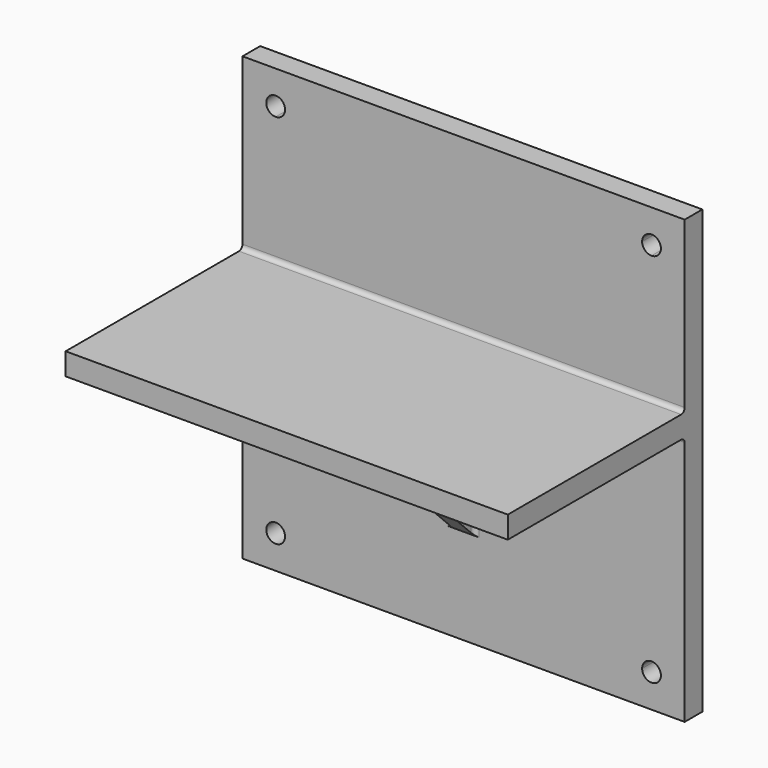
from build123d import *

# Parameters (mm, degrees)
F0_W         = 100
F0_H         = 10
F1_DEPTH     = 200
F2_W         = 10
F2_H         = 70
F3_DEPTH     = 70
F5_DEPTH     = 70
F7_DEPTH     = 20
F8_T1_DEPTH  = 200
F8_T3_DEPTH  = 93
F8_T5_DEPTH  = 93
F8_S9_W      = 2
F8_S9_H      = 2
F8_T10_DEPTH = 2
F8_S15_W     = 2
F8_S15_H     = 2
F8_T16_DEPTH = 2
F8_T22_DEPTH = 73
F8_T27_DEPTH = 73
F8_T32_DEPTH = 73
F8_T37_DEPTH = 73


# Not quite as in the source:
# - a fillet or chamfer that OpenCascade refuses, or shapes differently, is made with other operations: its cross-section is extruded or revolved along the edge and cut away or added


with BuildPart() as f1:
    # F0 (on Right) → F1 (new body)
    with BuildSketch(Plane.YZ):
        Polygon((5, -100), (5, 100), (-5, 100), (-5, 23.2), (-5, 13.2), (-5, -100), align=None)
        with Locations((-55, 18.2)):
            Rectangle(F0_W, F0_H)
    extrude(amount=F1_DEPTH)

    # F2 (on face) → F3 (join)
    with BuildSketch(Plane.XZ.offset(5)):
        with Locations((100, -21.8)):
            Rectangle(F2_W, F2_H)
    extrude(amount=F3_DEPTH)

    # F4 (on face) → F5 (cut)
    with BuildSketch(Plane(origin=(95, 0, 0), x_dir=(0, -1, 0), z_dir=(-1, 0, 0))):
        Polygon((75, -56.8), (75, 13.2), (5, -56.8), align=None)
    extrude(amount=-F5_DEPTH, mode=Mode.SUBTRACT)

    # F6 (on face) → F7 (cut)
    with BuildSketch(Plane.XZ.offset(5)):
        with BuildLine():
            Line((15, 80.75), (15, 85))
            Line((15, 85), (19.25, 85))
            ThreePointArc((19.25, 85), (11.99479618, 88.00520382), (15, 80.75))
        make_face()
        with BuildLine():
            Line((19.25, 85), (15, 85))
            Line((15, 85), (15, 80.75))
            ThreePointArc((15, 80.75), (18.00520382, 81.99479618), (19.25, 85))
        make_face()
        with BuildLine():
            ThreePointArc((189.25, 85), (185, 89.25), (180.75, 85))
            Line((180.75, 85), (185, 85))
            Line((185, 85), (185, 80.75))
            ThreePointArc((185, 80.75), (188.00520382, 81.99479618), (189.25, 85))
        make_face()
        with BuildLine():
            Line((185, 85), (180.75, 85))
            ThreePointArc((180.75, 85), (181.99479618, 81.99479618), (185, 80.75))
            Line((185, 80.75), (185, 85))
        make_face()
        with BuildLine():
            ThreePointArc((189.25, -85), (188.00520382, -81.99479618), (185, -80.75))
            Line((185, -80.75), (185, -85))
            Line((185, -85), (180.75, -85))
            ThreePointArc((180.75, -85), (185, -89.25), (189.25, -85))
        make_face()
        with BuildLine():
            Line((185, -85), (185, -80.75))
            ThreePointArc((185, -80.75), (181.99479618, -81.99479618), (180.75, -85))
            Line((180.75, -85), (185, -85))
        make_face()
        with BuildLine():
            Line((15, -85), (15, -80.75))
            ThreePointArc((15, -80.75), (11.99479618, -88.00520382), (19.25, -85))
            Line((19.25, -85), (15, -85))
        make_face()
        with BuildLine():
            ThreePointArc((19.25, -85), (18.00520382, -81.99479618), (15, -80.75))
            Line((15, -80.75), (15, -85))
            Line((15, -85), (19.25, -85))
        make_face()
    extrude(amount=-F7_DEPTH, mode=Mode.SUBTRACT)

    # F8: fillet of radius 2 on 7 edges, made by hand

    # F8_s2 → F8_t1 (join)
    with BuildSketch(Plane.YZ):
        with BuildLine():
            ThreePointArc((-5, 25.2), (-5.5857864376, 23.7857864376), (-7, 23.2))
            Line((-7, 23.2), (-5, 23.2))
            Line((-5, 23.2), (-5, 25.2))
        make_face()
    extrude(amount=F8_T1_DEPTH)

    # F8_s4 → F8_t3 (join)
    with BuildSketch(Plane.YZ):
        with BuildLine():
            ThreePointArc((-5, 11.2), (-5.5857864376, 12.6142135624), (-7, 13.2))
            Line((-7, 13.2), (-5, 13.2))
            Line((-5, 13.2), (-5, 11.2))
        make_face()
    extrude(amount=F8_T3_DEPTH)

    # F8_s6 → F8_t5 (join)
    with BuildSketch(Plane.YZ.offset(107)):
        with BuildLine():
            ThreePointArc((-5, 11.2), (-5.5857864376, 12.6142135624), (-7, 13.2))
            Line((-7, 13.2), (-5, 13.2))
            Line((-5, 13.2), (-5, 11.2))
        make_face()
    extrude(amount=F8_T5_DEPTH)


with BuildPart() as f8_tool8:
    # F8_s9 → F8_t10 (new body)
    with BuildSketch(Plane.XZ.offset(7)):
        with Locations((94, 12.2)):
            Rectangle(F8_S9_W, F8_S9_H)
    extrude(amount=-F8_T10_DEPTH)

    # F8_s11 → F8_t12 (revolve, cut)
    with BuildSketch(Plane(origin=(93, -7, 11.2), x_dir=(-0.7071067812, 0, -0.7071067812), z_dir=(0.7071067812, 0, -0.7071067812))):
        with BuildLine():
            ThreePointArc((0, -2), (2, 0), (0, 2))
            Line((0, 2), (0, -2))
        make_face()
    revolve(axis=Axis((93, -7, 11.2), (0, 1, 0)), mode=Mode.SUBTRACT)


with BuildPart() as f1_1:
    add(f1.part)

    # F8_t7: union F8_tool8
    add(f8_tool8.part)


with BuildPart() as f8_tool14:
    # F8_s15 → F8_t16 (new body)
    with BuildSketch(Plane.YZ.offset(107)):
        with Locations((-6, 12.2)):
            Rectangle(F8_S15_W, F8_S15_H)
    extrude(amount=-F8_T16_DEPTH)

    # F8_s17 → F8_t18 (revolve, cut)
    with BuildSketch(Plane(origin=(107, -7, 11.2), x_dir=(0, -0.7071067812, -0.7071067812), z_dir=(0, 0.7071067812, -0.7071067812))):
        with BuildLine():
            ThreePointArc((0, -2), (2, 0), (0, 2))
            Line((0, 2), (0, -2))
        make_face()
    revolve(axis=Axis((107, -7, 11.2), (-1, 0, 0)), mode=Mode.SUBTRACT)


with BuildPart() as f1_2:
    add(f1_1.part)

    # F8_t13: union F8_tool14
    add(f8_tool14.part)


with BuildPart() as f8_tool20:
    # F8_s21 → F8_t22 (new body)
    with BuildSketch(Plane.XY.offset(-61.8)):
        with BuildLine():
            ThreePointArc((107, -5), (105.5857864376, -5.5857864376), (105, -7))
            Line((105, -7), (105, -5))
            Line((105, -5), (107, -5))
        make_face()
    extrude(amount=F8_T22_DEPTH)

    split(bisect_by=Plane(origin=(0, -30.9, -30.9), x_dir=(1, 0, 0), z_dir=(0, 0.7071067812, 0.7071067812)), keep=Keep.TOP)


with BuildPart() as f1_3:
    add(f1_2.part)

    # F8_t19: union F8_tool20
    add(f8_tool20.part)


with BuildPart() as f8_tool25:
    # F8_s26 → F8_t27 (new body)
    with BuildSketch(Plane.XY.offset(11.2)):
        with BuildLine():
            ThreePointArc((93, -5), (94.4142135624, -5.5857864376), (95, -7))
            Line((95, -7), (95, -5))
            Line((95, -5), (93, -5))
        make_face()
    extrude(amount=-F8_T27_DEPTH)

    split(bisect_by=Plane(origin=(0, -30.9, -30.9), x_dir=(1, 0, 0), z_dir=(0, 0.7071067812, 0.7071067812)), keep=Keep.TOP)


with BuildPart() as f1_4:
    add(f1_3.part)

    # F8_t24: union F8_tool25
    add(f8_tool25.part)


with BuildPart() as f8_tool30:
    # F8_s31 → F8_t32 (new body)
    with BuildSketch(Plane.XZ.offset(7)):
        with BuildLine():
            ThreePointArc((93, 13.2), (94.4142135624, 12.6142135624), (95, 11.2))
            Line((95, 11.2), (95, 13.2))
            Line((95, 13.2), (93, 13.2))
        make_face()
    extrude(amount=F8_T32_DEPTH)

    split(bisect_by=Plane(origin=(0, -30.9, -30.9), x_dir=(1, 0, 0), z_dir=(0, 0.7071067812, 0.7071067812)), keep=Keep.TOP)


with BuildPart() as f1_5:
    add(f1_4.part)

    # F8_t29: union F8_tool30
    add(f8_tool30.part)


with BuildPart() as f8_tool35:
    # F8_s36 → F8_t37 (new body)
    with BuildSketch(Plane.XZ.offset(7)):
        with BuildLine():
            ThreePointArc((107, 13.2), (105.5857864376, 12.6142135624), (105, 11.2))
            Line((105, 11.2), (105, 13.2))
            Line((105, 13.2), (107, 13.2))
        make_face()
    extrude(amount=F8_T37_DEPTH)

    split(bisect_by=Plane(origin=(0, -30.9, -30.9), x_dir=(1, 0, 0), z_dir=(0, 0.7071067812, 0.7071067812)), keep=Keep.TOP)


with BuildPart() as f1_6:
    add(f1_5.part)

    # F8_t34: union F8_tool35
    add(f8_tool35.part)


solid = f1_6.part
